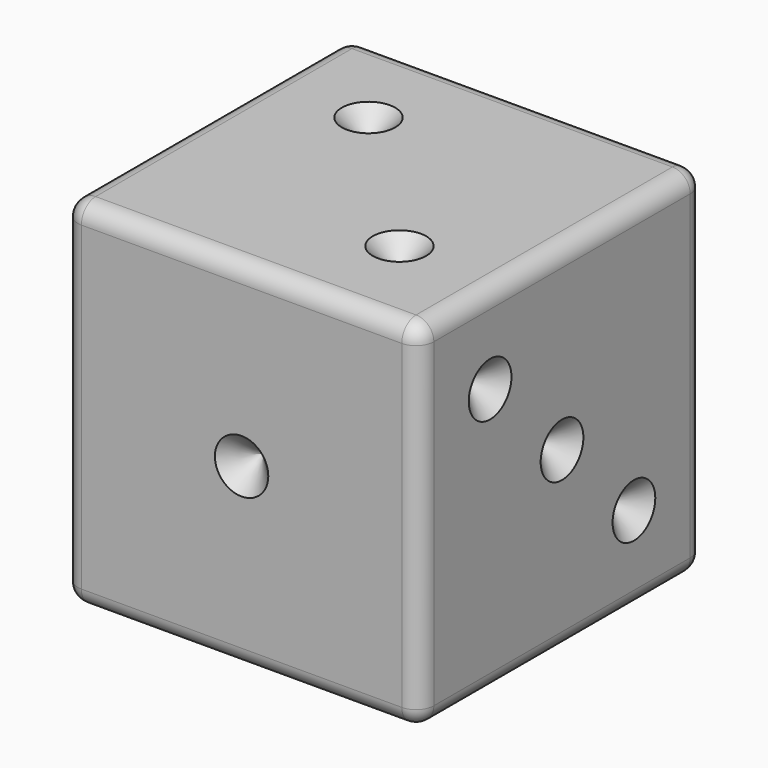
from build123d import *

# Parameters (mm, degrees)
F0_W      = 20
F0_H      = 20
F1_DEPTH  = 20
F2_R      = 1.5
F3_DEPTH  = 1.5
F4_R      = 1.5
F5_DEPTH  = 1.5
F6_R      = 1
F7_SIZE   = 1.49999
F8_R      = 1.5
F9_DEPTH  = 1.5
F10_SIZE  = 1.49999
F11_R     = 1.5
F12_DEPTH = 1.5
F13_SIZE  = 1.49999
F14_R     = 1.5
F15_DEPTH = 1.5
F16_SIZE  = 1.49999
F17_R     = 1.5
F18_DEPTH = 1.5
F19_SIZE  = 1.49999


# Not quite as in the source:
# - a fillet or chamfer is up to 0.001 mm smaller than in the source, because OpenCascade refuses the exact size


with BuildPart() as f1:
    # F0 (on Top) → F1 (new body)
    with BuildSketch(Plane.XY):
        with Locations((10, 10)):
            Rectangle(F0_W, F0_H)
    extrude(amount=F1_DEPTH)

    # F2 (on face) → F3 (cut)
    with BuildSketch(Plane.XZ):
        with Locations((10, 10)):
            Circle(F2_R)
    extrude(amount=-F3_DEPTH, mode=Mode.SUBTRACT)

    # F4 (on face) → F5 (cut)
    with BuildSketch(Plane.XY.offset(20)):
        with Locations((14.3431457505, 5.6568542495)):
            Circle(F4_R)
        with Locations((5.6568542495, 14.3431457505)):
            Circle(F4_R)
    extrude(amount=-F5_DEPTH, mode=Mode.SUBTRACT)

    # F6
    f6_edges = [f1.edges().sort_by_distance(p)[0] for p in [
        (0, 10, 20),
        (10, 20, 20),
        (20, 10, 20),
        (20, 10, 0),
        (10, 0, 20),
        (10, 0, 0),
        (0, 0, 10),
        (20, 0, 10),
        (20, 20, 10),
        (10, 20, 0),
        (0, 10, 0),
        (0, 20, 10),
    ]]
    fillet(f6_edges, radius=F6_R)

    # F7 (size 1.5 in the source; OpenCascade refuses exactly that, so slightly less here)
    f7_edges = [f1.edges().sort_by_distance(p)[0] for p in [
        (12.843146, 5.656854, 18.5),
        (4.156854, 14.343146, 18.5),
        (8.5, 1.5, 10),
    ]]
    chamfer(f7_edges, length=F7_SIZE)

    # F8 (on face) → F9 (cut)
    with BuildSketch(Plane.YZ.offset(20)):
        with Locations((15.0502525317, 4.9497474683)):
            Circle(F8_R)
        with Locations((4.9497474683, 15.0502525317)):
            Circle(F8_R)
        with Locations((10, 10)):
            Circle(F8_R)
    extrude(amount=-F9_DEPTH, mode=Mode.SUBTRACT)

    # F10 (size 1.5 in the source; OpenCascade refuses exactly that, so slightly less here)
    f10_edges = [f1.edges().sort_by_distance(p)[0] for p in [
        (18.5, 3.449747, 15.050253),
        (18.5, 8.5, 10),
        (18.5, 13.550253, 4.949747),
    ]]
    chamfer(f10_edges, length=F10_SIZE)

    # F11 (on face) → F12 (cut)
    with BuildSketch(Plane(origin=(0, 0, 0), x_dir=(0, -1, 0), z_dir=(-1, 0, 0))):
        with Locations((-14.3431457505, 14.3431457505)):
            Circle(F11_R)
        with Locations((-14.3431457505, 5.6568542495)):
            Circle(F11_R)
        with Locations((-5.6568542495, 14.3431457505)):
            Circle(F11_R)
        with Locations((-5.6568542495, 5.6568542495)):
            Circle(F11_R)
    extrude(amount=-F12_DEPTH, mode=Mode.SUBTRACT)

    # F13 (size 1.5 in the source; OpenCascade refuses exactly that, so slightly less here)
    f13_edges = [f1.edges().sort_by_distance(p)[0] for p in [
        (1.5, 15.843146, 14.343146),
        (1.5, 15.843146, 5.656854),
    ]]
    chamfer(f13_edges, length=F13_SIZE)

    # F14 (on face) → F15 (cut)
    with BuildSketch(Plane(origin=(0, 0, 0), x_dir=(1, 0, 0), z_dir=(0, 0, -1))):
        with Locations((4.9497474683, -15.0502525317)):
            Circle(F14_R)
        with Locations((15.0502525317, -15.0502525317)):
            Circle(F14_R)
        with Locations((15.0502525317, -4.9497474683)):
            Circle(F14_R)
        with Locations((4.9497474683, -4.9497474683)):
            Circle(F14_R)
        with Locations((10, -10)):
            Circle(F14_R)
    extrude(amount=-F15_DEPTH, mode=Mode.SUBTRACT)

    # F16 (size 1.5 in the source; OpenCascade refuses exactly that, so slightly less here)
    f16_edges = [f1.edges().sort_by_distance(p)[0] for p in [
        (3.449747, 4.949747, 1.5),
        (13.550253, 4.949747, 1.5),
        (8.5, 10, 1.5),
        (3.449747, 15.050253, 1.5),
        (13.550253, 15.050253, 1.5),
    ]]
    chamfer(f16_edges, length=F16_SIZE)

    # F17 (on face) → F18 (cut)
    with BuildSketch(Plane(origin=(0, 20, 0), x_dir=(-1, 0, 0), z_dir=(0, 1, 0))):
        with Locations((-5.1666666667, 9.6666666667)):
            Circle(F17_R)
        with Locations((-5.1666666667, 14.8333333333)):
            Circle(F17_R)
        with Locations((-14.8333333333, 4.5)):
            Circle(F17_R)
        with Locations((-5.1666666667, 4.5)):
            Circle(F17_R)
        with Locations((-14.8333333333, 14.8333333333)):
            Circle(F17_R)
        with Locations((-14.8333333333, 9.6666666667)):
            Circle(F17_R)
    extrude(amount=-F18_DEPTH, mode=Mode.SUBTRACT)

    # F19 (size 1.5 in the source; OpenCascade refuses exactly that, so slightly less here)
    f19_edges = [f1.edges().sort_by_distance(p)[0] for p in [
        (16.333333, 18.5, 14.833333),
        (6.666667, 18.5, 14.833333),
        (6.666667, 18.5, 9.666667),
        (6.666667, 18.5, 4.5),
        (16.333333, 18.5, 4.5),
        (16.333333, 18.5, 9.666667),
    ]]
    chamfer(f19_edges, length=F19_SIZE)


solid = f1.part
